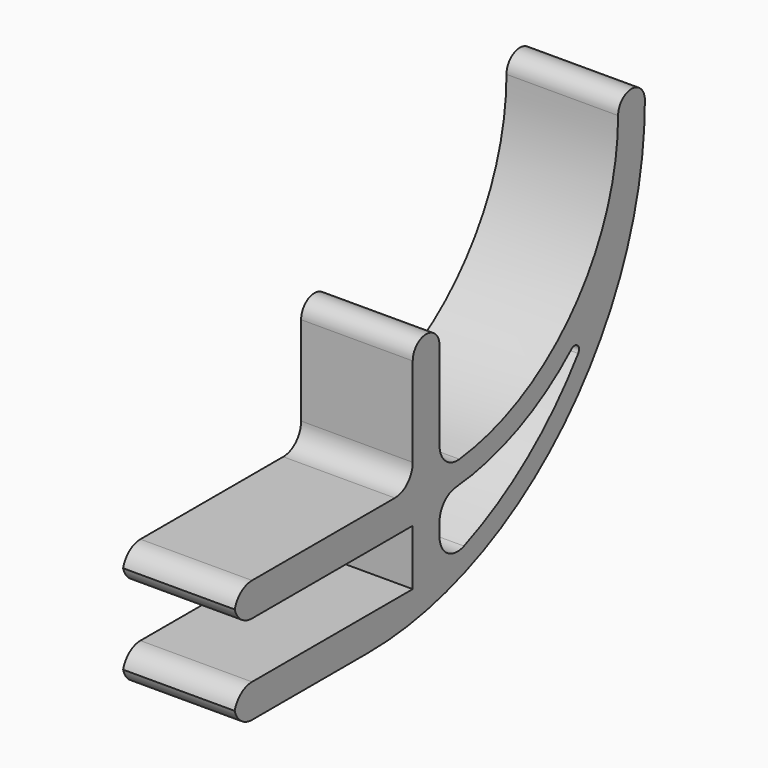
from build123d import *

# Parameters (mm, degrees)
F1_DEPTH    = 10
F2_T1_DEPTH = 10
F2_T3_DEPTH = 20


# Not quite as in the source:
# - a fillet or chamfer that OpenCascade refuses, or shapes differently, is made with other operations: its cross-section is extruded or revolved along the edge and cut away or added
# - a feature names something its author has since deleted; it is built from what else it names


with BuildPart() as f1:
    # F0 (on Right) → F1 (new body)
    with BuildSketch(Plane.YZ):
        with BuildLine():
            Line((20, 0), (0, 0))
            Line((0, 0), (0, -3))
            Line((0, -3), (15, -3))
            ThreePointArc((15, -3), (36.9203102168, 6.0796897832), (46, 28))
            ThreePointArc((46, 28), (44.5, 29.5), (43, 28))
            ThreePointArc((43, 28), (37.1421356237, 13.8578643763), (23, 8))
            Line((23, 8), (23, 18))
            ThreePointArc((23, 18), (21.5, 19.5), (20, 18))
            Line((20, 18), (20, 8))
            Line((20, 8), (0, 8))
            Line((0, 8), (0, 5))
            Line((0, 5), (20, 5))
            Line((20, 5), (20, 0))
        make_face()
        with BuildLine():
            Line((23, 0.1252802705), (23, 6))
            ThreePointArc((23, 6), (30.9268806632, 7.4777057094), (37.7888888889, 11.712312459))
            ThreePointArc((37.7888888889, 11.712312459), (38.4580316617, 11.7150853421), (38.5307017544, 11.0498945447))
            ThreePointArc((38.5307017544, 11.0498945447), (31.6848160775, 4.2804529457), (23, 0.1252802705))
        make_face(mode=Mode.SUBTRACT)
    extrude(amount=F1_DEPTH)

    # F2: fillet of radius 2 on 8 edges, made by hand

    # F2_s2 → F2_t1 (join)
    with BuildSketch(Plane.YZ):
        with BuildLine():
            ThreePointArc((20, 10), (19.4142135624, 8.5857864376), (18, 8))
            Line((18, 8), (20, 8))
            Line((20, 8), (20, 10))
        make_face()
        with BuildLine():
            ThreePointArc((25.2222222222, 8.1238402), (23.6666666667, 8.620744195), (23, 10.11145618))
            Line((23, 10.11145618), (23, 8))
            ThreePointArc((23, 8), (24.1128351181, 8.0309840503), (25.2222222222, 8.1238402))
        make_face()
        with BuildLine():
            ThreePointArc((23, 4.0834785138), (23.5280398556, 5.4374849146), (24.8333333333, 6.076521971))
            ThreePointArc((24.8333333333, 6.076521971), (23.9174648117, 6.0191388176), (23, 6))
            Line((23, 6), (23, 4.0834785138))
        make_face()
        with BuildLine():
            ThreePointArc((25.7407407407, 1.0623592655), (23.8778327846, 1.2646093225), (23, 2.920127592))
            Line((23, 2.920127592), (23, 0.1252802705))
            ThreePointArc((23, 0.1252802705), (24.3820770695, 0.5595803629), (25.7407407407, 1.0623592655))
        make_face()
    extrude(amount=F2_T1_DEPTH)

    # F2_s4 → F2_t3 (cut)
    with BuildSketch(Plane.YZ.offset(-5)):
        with BuildLine():
            ThreePointArc((2, 8), (0.5857864376, 7.4142135624), (0, 6))
            Line((0, 6), (0, 8))
            Line((0, 8), (2, 8))
        make_face()
        with BuildLine():
            ThreePointArc((0, 7), (0.5857864376, 5.5857864376), (2, 5))
            Line((2, 5), (0, 5))
            Line((0, 5), (0, 7))
        make_face()
        with BuildLine():
            ThreePointArc((2, 0), (0.5857864376, -0.5857864376), (0, -2))
            Line((0, -2), (0, 0))
            Line((0, 0), (2, 0))
        make_face()
        with BuildLine():
            ThreePointArc((0, -1), (0.5857864376, -2.4142135624), (2, -3))
            Line((2, -3), (0, -3))
            Line((0, -3), (0, -1))
        make_face()
    extrude(amount=F2_T3_DEPTH, mode=Mode.SUBTRACT)


solid = f1.part
